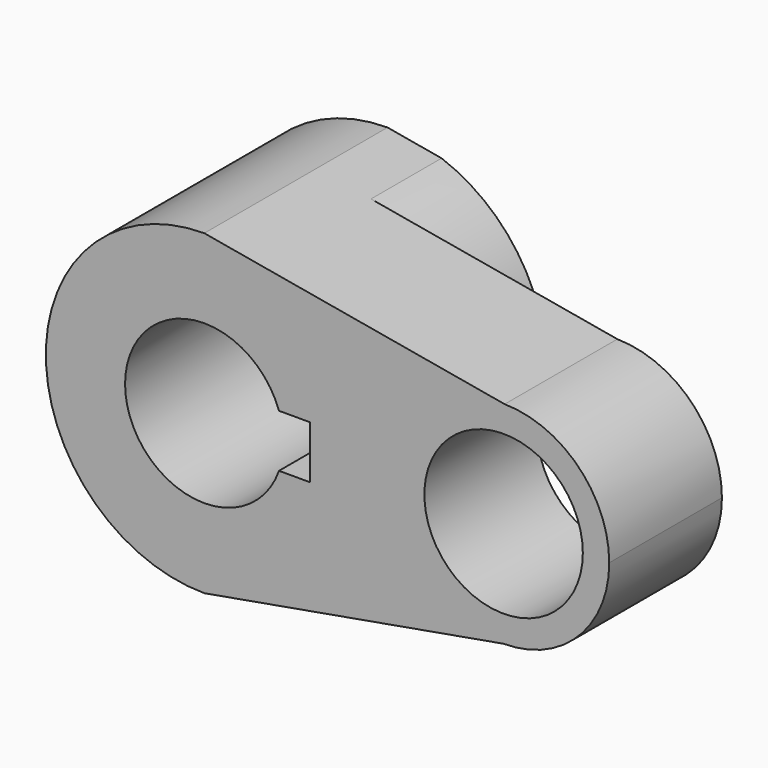
from build123d import *

# Parameters (mm, degrees)
F0_R     = 14.2875
F1_DEPTH = 25.4
F2_DEPTH = 15.89601


with BuildPart() as f1:
    # F0 (on Front) → F1 (new body)
    with BuildSketch(Plane.XZ):
        with BuildLine():
            Line((9.7499238233, 26.8601863441), (0, 28.575))
            ThreePointArc((0, 28.575), (-28.575, 0), (0, -28.575))
            Line((0, -28.575), (9.7818449028, -26.8485779008))
            ThreePointArc((9.7818449028, -26.8485779008), (23.4099000756, -16.3861894122), (28.575, 0))
            ThreePointArc((28.575, 0), (23.4001570321, 16.4000998739), (9.7499238233, 26.8601863441))
        make_face()
        with BuildLine():
            ThreePointArc((-13.4703841816, 4.7625), (0, 14.2875), (13.4703841816, 4.7625))
            Line((13.4703841816, 4.7625), (19.05, 4.7625))
            Line((19.05, 4.7625), (19.05, -4.7625))
            Line((19.05, -4.7625), (13.4703841816, -4.7625))
            ThreePointArc((13.4703841816, -4.7625), (0, -14.2875), (-13.4703841816, -4.7625))
            Line((-13.4703841816, -4.7625), (-19.05, -4.7625))
            Line((-19.05, -4.7625), (-19.05, 4.7625))
            Line((-19.05, 4.7625), (-13.4703841816, 4.7625))
        make_face(mode=Mode.SUBTRACT)
        with BuildLine():
            Line((54.1615282252, 19.0490867818), (9.7499238233, 26.8601863441))
            ThreePointArc((9.7499238233, 26.8601863441), (23.4001570321, 16.4000998739), (28.575, 0))
            ThreePointArc((28.575, 0), (23.4099000756, -16.3861894122), (9.7818449028, -26.8485779008))
            Line((9.7818449028, -26.8485779008), (53.9683106658, -19.0499988255))
            ThreePointArc((53.9683106658, -19.0499988255), (34.9252449744, 0.096609856), (54.1615282252, 19.0490867818))
        make_face()
        with BuildLine():
            ThreePointArc((73.025, 0), (67.5111712218, 13.4042742681), (54.1615282252, 19.0490867818))
            ThreePointArc((54.1615282252, 19.0490867818), (34.9252449744, 0.096609856), (53.9683106658, -19.0499988255))
            ThreePointArc((53.9683106658, -19.0499988255), (67.4430189372, -13.4727490108), (73.025, 0))
        make_face()
        with Locations((53.975, 0)):
            Circle(F0_R, mode=Mode.SUBTRACT)
        with BuildLine():
            ThreePointArc((-13.4703841816, -4.7625), (-14.2875, 0), (-13.4703841816, 4.7625))
            Line((-13.4703841816, 4.7625), (-19.05, 4.7625))
            Line((-19.05, 4.7625), (-19.05, -4.7625))
            Line((-19.05, -4.7625), (-13.4703841816, -4.7625))
        make_face()
    extrude(amount=F1_DEPTH)

    # F0 (on Front) → F2 (join)
    with BuildSketch(Plane.XZ):
        with BuildLine():
            Line((9.7499238233, 26.8601863441), (0, 28.575))
            ThreePointArc((0, 28.575), (-28.575, 0), (0, -28.575))
            Line((0, -28.575), (9.7818449028, -26.8485779008))
            ThreePointArc((9.7818449028, -26.8485779008), (23.4099000756, -16.3861894122), (28.575, 0))
            ThreePointArc((28.575, 0), (23.4001570321, 16.4000998739), (9.7499238233, 26.8601863441))
        make_face()
        with BuildLine():
            ThreePointArc((-13.4703841816, 4.7625), (0, 14.2875), (13.4703841816, 4.7625))
            Line((13.4703841816, 4.7625), (19.05, 4.7625))
            Line((19.05, 4.7625), (19.05, -4.7625))
            Line((19.05, -4.7625), (13.4703841816, -4.7625))
            ThreePointArc((13.4703841816, -4.7625), (0, -14.2875), (-13.4703841816, -4.7625))
            Line((-13.4703841816, -4.7625), (-19.05, -4.7625))
            Line((-19.05, -4.7625), (-19.05, 4.7625))
            Line((-19.05, 4.7625), (-13.4703841816, 4.7625))
        make_face(mode=Mode.SUBTRACT)
        with BuildLine():
            ThreePointArc((-13.4703841816, -4.7625), (-14.2875, 0), (-13.4703841816, 4.7625))
            Line((-13.4703841816, 4.7625), (-19.05, 4.7625))
            Line((-19.05, 4.7625), (-19.05, -4.7625))
            Line((-19.05, -4.7625), (-13.4703841816, -4.7625))
        make_face()
    extrude(amount=-F2_DEPTH)


solid = f1.part
